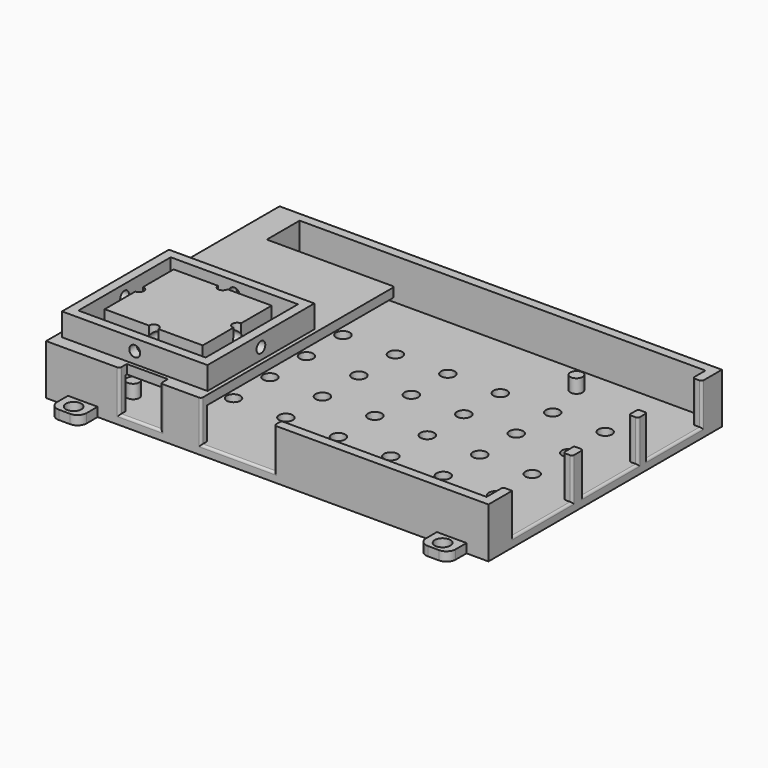
from build123d import *

# Parameters (mm, degrees)
F0_W         = 6
F0_H         = 60
F0_W_2       = 89
F0_H_2       = 2
F0_W_3       = 2
F1_DEPTH     = 11
F0_R         = 1.35
F2_DEPTH     = 2
F3_DEPTH     = 5
F4_W         = 9
F4_H         = 9
F4_W_2       = 16
F5_DEPTH     = 2
F6_W         = 16.5
F6_H         = 9
F6_W_2       = 15
F7_DEPTH     = 2
F8_DEPTH     = 8
F9_W         = 51
F9_H         = 2
F10_DEPTH    = 28
F11_W        = 6.5
F11_H        = 5
F11_R        = 1.5
F11_H_2      = 2
F11_H_3      = 1.5
F12_DEPTH    = 2
F13_R        = 2
F14_W        = 31.9
F14_H        = 29.3
F14_W_2      = 27.9
F14_H_2      = 25.3
F15_DEPTH    = 5
F18_R        = 1.5
F19_DEPTH    = 2
F20_R        = 0.5
F21_D        = 3.4
F22_D        = 2.4
F22_ON_F16_D = 2.4


with BuildPart() as f1:
    # F0 (on Top) → F1 (new body)
    with BuildSketch(Plane.XY):
        with Locations((-37.083922714, 20.717205769)):
            Rectangle(F0_W, F0_H)
        with Locations((10.416077286, 51.717205769)):
            Rectangle(F0_W_2, F0_H_2)
        with Locations((10.416077286, -10.282794231)):
            Rectangle(F0_W_2, F0_H_2)
        with Locations((-37.083922714, -10.282794231)):
            Rectangle(F0_W, F0_H_2)
        with Locations((-37.083922714, 51.717205769)):
            Rectangle(F0_W, F0_H_2)
        with Locations((55.916077286, 51.717205769)):
            Rectangle(F0_W_3, F0_H_2)
        with Locations((55.916077286, 20.717205769)):
            Rectangle(F0_W_3, F0_H)
        with Locations((55.916077286, -10.282794231)):
            Rectangle(F0_W_3, F0_H_2)
    extrude(amount=F1_DEPTH)

    # F0 (on Top) → F2 (join)
    with BuildSketch(Plane.XY):
        with Locations((10.416077286, 20.717205769)):
            Rectangle(F0_W_2, F0_H)
        with Locations((-26.583922714, -4.282794231)):
            Circle(F0_R, mode=Mode.SUBTRACT)
        with Locations((31.416077286, -4.282794231)):
            Circle(F0_R, mode=Mode.SUBTRACT)
        with Locations((-26.583922714, 44.717205769)):
            Circle(F0_R, mode=Mode.SUBTRACT)
        with Locations((31.416077286, 44.717205769)):
            Circle(F0_R, mode=Mode.SUBTRACT)
    extrude(amount=F2_DEPTH)

    # F0 (on Top) → F3 (join)
    with BuildSketch(Plane.XY):
        with Locations((-26.583922714, -4.282794231)):
            Circle(F0_R)
        with Locations((31.416077286, -4.282794231)):
            Circle(F0_R)
        with Locations((31.416077286, 44.717205769)):
            Circle(F0_R)
        with Locations((-26.583922714, 44.717205769)):
            Circle(F0_R)
    extrude(amount=F3_DEPTH)

    # F4 (on face) → F5 (cut, through all)
    with BuildSketch(Plane.XZ.offset(11.282794231)):
        with Locations((-19.483922714, 6.5)):
            Rectangle(F4_W, F4_H)
        with Locations((1.916077286, 6.5)):
            Rectangle(F4_W_2, F4_H)
    extrude(amount=-F5_DEPTH, mode=Mode.SUBTRACT)

    # F6 (on face) → F7 (cut, through all)
    with BuildSketch(Plane.YZ.offset(56.916077286)):
        with Locations((3.467205769, 6.5)):
            Rectangle(F6_W, F6_H)
        with Locations((22.217205769, 6.5)):
            Rectangle(F6_W_2, F6_H)
        with Locations((39.717205769, 6.5)):
            Rectangle(F6_W_2, F6_H)
    extrude(amount=-F7_DEPTH, mode=Mode.SUBTRACT)

    # F0 (on Top) → F8 (join)
    with BuildSketch(Plane.XY):
        with Locations((-37.083922714, 20.717205769)):
            Rectangle(F0_W, F0_H)
        with Locations((-37.083922714, 51.717205769)):
            Rectangle(F0_W, F0_H_2)
        with Locations((-37.083922714, -10.282794231)):
            Rectangle(F0_W, F0_H_2)
    extrude(amount=F8_DEPTH)

    # F9 (on face) → F10 (join)
    with BuildSketch(Plane.YZ.offset(-34.083922714)):
        with Locations((16.217205769, 10)):
            Rectangle(F9_W, F9_H)
    extrude(amount=F10_DEPTH)

    # F11 (on face) → F12 (join)
    with BuildSketch(Plane(origin=(0, 0, 0), x_dir=(1, 0, 0), z_dir=(0, 0, -1))):
        with Locations((48.866077286, 13.782794231)):
            Rectangle(F11_W, F11_H)
        with Locations((48.866077286, 13.782794231)):
            Circle(F11_R, mode=Mode.SUBTRACT)
        with Locations((48.866077286, -55.217205769)):
            Rectangle(F11_W, F11_H)
        with Locations((48.866077286, -55.217205769)):
            Circle(F11_R, mode=Mode.SUBTRACT)
        with Locations((-32.033922714, -55.217205769)):
            Rectangle(F11_W, F11_H)
        with Locations((-32.033922714, -55.217205769)):
            Circle(F11_R, mode=Mode.SUBTRACT)
        with Locations((-32.033922714, 13.782794231)):
            Rectangle(F11_W, F11_H)
        with Locations((-32.033922714, 13.782794231)):
            Circle(F11_R, mode=Mode.SUBTRACT)
        with Locations((48.866077286, 10.282794231)):
            Rectangle(F11_W, F11_H_2)
        with Locations((48.866077286, -51.717205769)):
            Rectangle(F11_W, F11_H_2)
        with Locations((-32.033922714, -51.967205769)):
            Rectangle(F11_W, F11_H_3)
        with Locations((-32.033922714, 10.532794231)):
            Rectangle(F11_W, F11_H_3)
        with Locations((-32.033922714, 13.782794231)):
            Circle(F11_R)
        with Locations((-32.033922714, -55.217205769)):
            Circle(F11_R)
        with Locations((48.866077286, -55.217205769)):
            Circle(F11_R)
        with Locations((48.866077286, 13.782794231)):
            Circle(F11_R)
    extrude(amount=-F12_DEPTH)

    # F13
    f13_edges = [f1.edges().sort_by_distance(p)[0] for p in [
        (-28.783923, 57.717206, 1),
        (-35.283923, 57.717206, 1),
        (-35.283923, -16.282794, 1),
        (-28.783923, -16.282794, 1),
        (45.616077, -16.282794, 1),
        (52.116077, -16.282794, 1),
        (52.116077, 57.717206, 1),
        (45.616077, 57.717206, 1),
    ]]
    fillet(f13_edges, radius=F13_R)

    # F14 (on face) → F15 (join)
    with BuildSketch(Plane.XY.offset(11)):
        with Locations((-22.883922714, 6.167205769)):
            Rectangle(F14_W, F14_H)
        with Locations((-22.883922714, 6.167205769)):
            Rectangle(F14_W_2, F14_H_2, mode=Mode.SUBTRACT)
        with BuildLine():
            ThreePointArc((-23.933922714, -3.282794231), (-22.883922714, -2.232794231), (-21.833922714, -3.282794231))
            Line((-21.833922714, -3.282794231), (-12.133922714, -3.282794231))
            Line((-12.133922714, -3.282794231), (-12.133922714, 5.117205769))
            ThreePointArc((-12.133922714, 5.117205769), (-13.183922714, 6.167205769), (-12.133922714, 7.217205769))
            Line((-12.133922714, 7.217205769), (-12.133922714, 15.617205769))
            Line((-12.133922714, 15.617205769), (-21.833922714, 15.617205769))
            ThreePointArc((-21.833922714, 15.617205769), (-22.883922714, 14.567205769), (-23.933922714, 15.617205769))
            Line((-23.933922714, 15.617205769), (-33.633922714, 15.617205769))
            Line((-33.633922714, 15.617205769), (-33.633922714, 7.217205769))
            ThreePointArc((-33.633922714, 7.217205769), (-32.8914605937, 6.9096678892), (-32.583922714, 6.167205769))
            ThreePointArc((-32.583922714, 6.167205769), (-32.8914605937, 5.4247436487), (-33.633922714, 5.117205769))
            Line((-33.633922714, 5.117205769), (-33.633922714, -3.282794231))
            Line((-33.633922714, -3.282794231), (-23.933922714, -3.282794231))
        make_face()
    extrude(amount=F15_DEPTH)

    # F18 (on face) → F19 (cut, through all)
    with BuildSketch(Plane.XY.offset(2)):
        with Locations((44.916077286, 5.717205769)):
            Circle(F18_R)
        with Locations((44.916077286, 15.717205769)):
            Circle(F18_R)
        with Locations((44.916077286, 25.717205769)):
            Circle(F18_R)
        with Locations((44.916077286, 35.717205769)):
            Circle(F18_R)
        with Locations((33.416077286, 35.717205769)):
            Circle(F18_R)
        with Locations((33.416077286, 25.717205769)):
            Circle(F18_R)
        with Locations((33.416077286, 15.717205769)):
            Circle(F18_R)
        with Locations((33.416077286, 5.717205769)):
            Circle(F18_R)
        with Locations((21.916077286, 5.717205769)):
            Circle(F18_R)
        with Locations((21.916077286, 15.717205769)):
            Circle(F18_R)
        with Locations((21.916077286, 25.717205769)):
            Circle(F18_R)
        with Locations((21.916077286, 35.717205769)):
            Circle(F18_R)
        with Locations((10.416077286, 35.717205769)):
            Circle(F18_R)
        with Locations((10.416077286, 25.717205769)):
            Circle(F18_R)
        with Locations((10.416077286, 15.717205769)):
            Circle(F18_R)
        with Locations((10.416077286, 5.717205769)):
            Circle(F18_R)
        with Locations((-1.083922714, 5.717205769)):
            Circle(F18_R)
        with Locations((-1.083922714, 15.717205769)):
            Circle(F18_R)
        with Locations((-1.083922714, 25.717205769)):
            Circle(F18_R)
        with Locations((-1.083922714, 35.717205769)):
            Circle(F18_R)
        with Locations((-12.583922714, 35.717205769)):
            Circle(F18_R)
        with Locations((-12.583922714, 25.717205769)):
            Circle(F18_R)
        with Locations((-12.583922714, 15.717205769)):
            Circle(F18_R)
        with Locations((-12.583922714, 5.717205769)):
            Circle(F18_R)
        with Locations((-24.083922714, 15.717205769)):
            Circle(F18_R)
        with Locations((-24.083922714, 25.717205769)):
            Circle(F18_R)
        with Locations((-24.083922714, 35.717205769)):
            Circle(F18_R)
        with Locations((-24.083922714, 5.717205769)):
            Circle(F18_R)
    extrude(amount=-F19_DEPTH, mode=Mode.SUBTRACT)

    # F20
    f20_edges = [f1.edges().sort_by_distance(p)[0] for p in [
        (56.916077, 11.717206, 6.5),
        (56.916077, 14.717206, 6.5),
        (56.916077, 29.717206, 6.5),
        (56.916077, 32.217206, 6.5),
        (56.916077, 47.217206, 6.5),
        (9.916077, -11.282794, 6.5),
        (-6.083923, -11.282794, 6.5),
        (-14.983923, -11.282794, 6.5),
        (-23.983923, -11.282794, 6.5),
        (9.916077, -9.282794, 6.5),
        (-6.083923, -9.282794, 5.5),
        (54.916077, -4.782794, 6.5),
        (54.916077, 11.717206, 6.5),
        (54.916077, 29.717206, 6.5),
        (54.916077, 32.217206, 6.5),
        (54.916077, 47.217206, 6.5),
        (-23.983923, -9.282794, 5.5),
        (-14.983923, -9.282794, 5.5),
        (1.916077, -11.282794, 2),
        (56.916077, 3.467206, 2),
        (56.916077, 22.217206, 2),
        (56.916077, 39.717206, 2),
        (-19.483923, -11.282794, 2),
        (-6.083923, 41.717206, 10),
    ]]
    fillet(f20_edges, radius=F20_R)

    # F21 (through all)
    with Locations(Plane(origin=(0, 0, 0), x_dir=(1, 0, 0), z_dir=(0, 0, -1))):
        with Locations((48.866077286, 13.782794231), (-32.033922714, 13.782794231), (48.866077286, -55.217205769), (-32.033922714, -55.217205769)):
            Hole(F21_D / 2)

    # F22 (through all)
    with Locations(Plane(origin=(0, 20.817205769, 0), x_dir=(-1, 0, 0), z_dir=(0, 1, 0))):
        with Locations((22.883922714, 13.5)):
            Hole(F22_D / 2)

    # F22 on F16 (through all)
    with Locations(Plane(origin=(-40.083922714, 0, 0), x_dir=(0, -1, 0), z_dir=(-1, 0, 0))):
        with Locations((-6.167205769, 13.5)):
            Hole(F22_ON_F16_D / 2)


solid = f1.part
